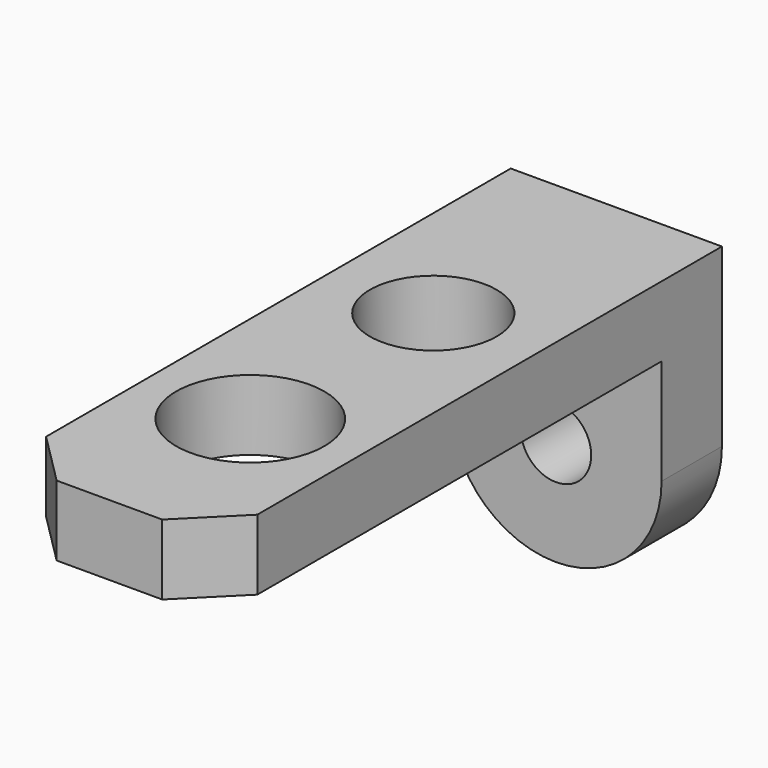
from build123d import *

# Parameters (mm, degrees)
F0_W     = 152.4
F0_H     = 457.2
F1_DEPTH = 50.8
F2_W     = 152.4
F2_H     = 54.4068123519
F3_DEPTH = 152.4
F4_R     = 76.19999
F5_R     = 45.72
F5_R_2   = 53.4879372825
F6_DEPTH = 50.801
F7_R     = 25.4
F8_DEPTH = 54.4078123519
F9_SIZE  = 38.1


# Not quite as in the source:
# - a fillet or chamfer is up to 0.001 mm smaller than in the source, because OpenCascade refuses the exact size


with BuildPart() as f1:
    # F0 (on Top) → F1 (new body)
    with BuildSketch(Plane.XY):
        with Locations((39.8436626315, 216.4812246025)):
            Rectangle(F0_W, F0_H)
    extrude(amount=F1_DEPTH)

    # F2 (on face) → F3 (join)
    with BuildSketch(Plane(origin=(0, 0, 0), x_dir=(1, 0, 0), z_dir=(0, 0, -1))):
        with Locations((39.8436626315, -417.8778184265)):
            Rectangle(F2_W, F2_H)
    extrude(amount=F3_DEPTH)

    # F4 (radius 76.2 in the source; OpenCascade refuses exactly that, so slightly less here)
    f4_edges = [f1.edges().sort_by_distance(p)[0] for p in [
        (116.043663, 417.877818, -152.4),
        (-36.356337, 417.877818, -152.4),
    ]]
    fillet(f4_edges, radius=F4_R)

    # F5 (on face) → F6 (cut, through all)
    with BuildSketch(Plane(origin=(0, 0, 0), x_dir=(1, 0, 0), z_dir=(0, 0, -1))):
        with Locations((39.8436626315, -279.9812246025)):
            Circle(F5_R)
        with Locations((39.8436626315, -114.8812246025)):
            Circle(F5_R_2)
    extrude(amount=-F6_DEPTH, mode=Mode.SUBTRACT)

    # F7 (on face) → F8 (cut, through all)
    with BuildSketch(Plane.XZ.offset(-390.6744122505)):
        with Locations((39.8436626315, -76.2)):
            Circle(F7_R)
    extrude(amount=-F8_DEPTH, mode=Mode.SUBTRACT)

    # F9
    f9_edges = [f1.edges().sort_by_distance(p)[0] for p in [
        (116.043663, -12.118775, 25.4),
        (-36.356337, -12.118775, 25.4),
    ]]
    chamfer(f9_edges, length=F9_SIZE)


solid = f1.part
